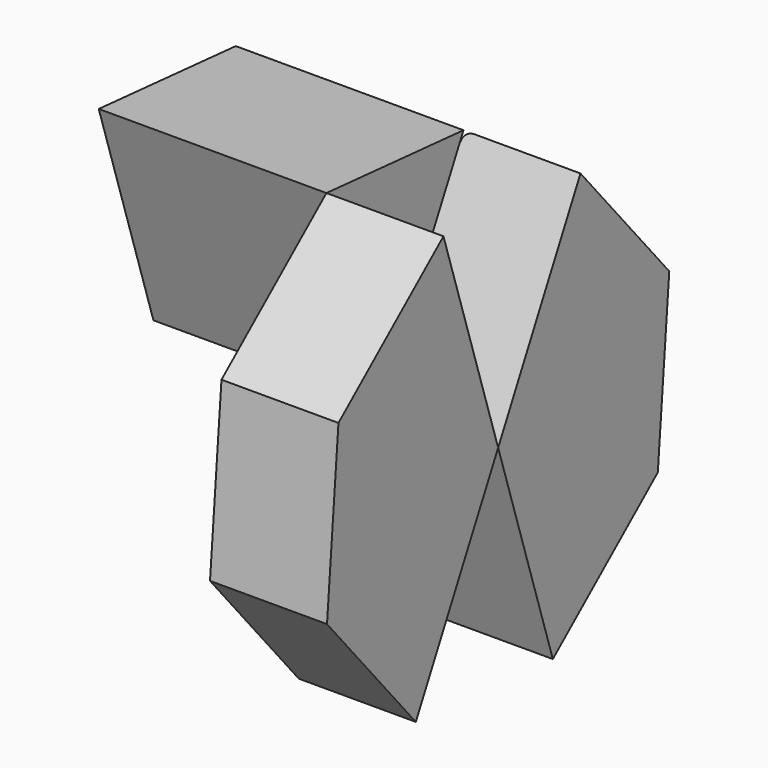
from build123d import *

# Parameters (mm, degrees)
F1_DEPTH     = 12.7
F2_DEPTH     = 25.4
F3_T1_DEPTH  = 25.0079243049
F3_T3_DEPTH  = 25.0079243049
F3_T5_DEPTH  = 25.0079243049
F4_T         = -2.54
F5_T4_DEPTH  = 36.4551670306
F5_T10_DEPTH = 39.8442718127
F5_T16_DEPTH = 39.8442718127
F5_T23_DEPTH = 36.4551670306
F5_T29_DEPTH = 39.8442718127
F5_T38_DEPTH = 36.4551670306
F5_T44_DEPTH = 39.8442718127
F5_T53_DEPTH = 39.8442718127
F5_T59_DEPTH = 39.8442718127


# Not quite as in the source:
# - a fillet or chamfer that OpenCascade refuses, or shapes differently, is made with other operations: its cross-section is extruded or revolved along the edge and cut away or added


with BuildPart() as f1:
    # F0 (on Right) → F1 (new body)
    with BuildSketch(Plane.YZ):
        Polygon((-7.4210610107, 23.220738357), (-21.6670241207, 11.1720589921), (-23.220738357, -7.4210610107), (-11.1720589921, -21.6670241207), (0, 0), align=None)
    extrude(amount=F1_DEPTH)


with BuildPart() as f1b:
    # F0 (on Right) → F1, piece 2 (new body)
    with BuildSketch(Plane.YZ):
        Polygon((23.220738357, 7.4210610107), (11.1720589921, 21.6670241207), (0, 0), (7.4210610107, -23.220738357), (21.6670241207, -11.1720589921), align=None)
    extrude(amount=F1_DEPTH)

    # F3: fillet of radius 1.27 on 3 edges, made by hand

    # F3_s2 → F3_t1 (cut)
    with BuildSketch(Plane(origin=(0, -9.5472026063, -8.074651194), x_dir=(1, 0, 0), z_dir=(0, 0.7635341894, 0.6457674052))):
        with BuildLine():
            add(Edge.make_bspline(
                [(1.27, 22.5221069513), (0, 22.5221069513), (0, 21.2521069513)],
                knots=[0, 0, 0, 1, 1, 1], degree=2, weights=[1, 1, 1]))
            Line((0, 21.2521069513), (0, 22.5221069513))
            Line((0, 22.5221069513), (1.27, 22.5221069513))
        make_face()
    extrude(amount=F3_T1_DEPTH, mode=Mode.SUBTRACT)

    # F3_s4 → F3_t3 (cut)
    with BuildSketch(Plane(origin=(0, -1.0412510893, -12.4605323193), x_dir=(1, 0, 0), z_dir=(0, 0.0832736917, 0.9965267143))):
        with BuildLine():
            add(Edge.make_bspline(
                [(1.27, 22.5221069513), (0, 22.5221069513), (0, 21.2521069513)],
                knots=[0, 0, 0, 1, 1, 1], degree=2, weights=[1, 1, 1]))
            Line((0, 21.2521069513), (0, 22.5221069513))
            Line((0, 22.5221069513), (1.27, 22.5221069513))
        make_face()
    extrude(amount=F3_T3_DEPTH, mode=Mode.SUBTRACT)

    # F3_s6 → F3_t5 (cut)
    with BuildSketch(Plane(origin=(0, 8.074651194, -9.5472026063), x_dir=(1, 0, 0), z_dir=(0, -0.6457674052, 0.7635341894))):
        with BuildLine():
            add(Edge.make_bspline(
                [(1.27, 22.5221069513), (0, 22.5221069513), (0, 21.2521069513)],
                knots=[0, 0, 0, 1, 1, 1], degree=2, weights=[1, 1, 1]))
            Line((0, 21.2521069513), (0, 22.5221069513))
            Line((0, 22.5221069513), (1.27, 22.5221069513))
        make_face()
    extrude(amount=F3_T5_DEPTH, mode=Mode.SUBTRACT)


with BuildPart() as f2:
    # F0 (on Right) → F2 (new body)
    with BuildSketch(Plane.YZ):
        Polygon((11.1720589921, 21.6670241207), (-7.4210610107, 23.220738357), (0, 0), align=None)
    extrude(amount=-F2_DEPTH)

    # F4
    f4_openings = [f2.faces().sort_by_distance(p)[0] for p in [
        (-25.4, 1.250333, 14.962587),
    ]]
    offset(amount=F4_T, openings=f4_openings)

    # F5: fillet of radius 5.08 on 3 edges, made by hand


with BuildPart() as f5_tool2:
    # F5_s3 → F5_t4 (new body)
    with BuildSketch(Plane(origin=(0, 18.1642739097, -1.5178781701), x_dir=(1, 0, 0), z_dir=(0, -0.9965267143, 0.0832736917))):
        with BuildLine():
            ThreePointArc((-25.4, 25.0621069513), (-23.9121024484, 21.4700045029), (-20.32, 19.9821069513))
            Line((-20.32, 19.9821069513), (-25.4, 19.9821069513))
            Line((-25.4, 19.9821069513), (-25.4, 25.0621069513))
        make_face()
    extrude(amount=F5_T4_DEPTH)

    split(bisect_by=Plane(origin=(0, 2.4194467666, 0.7732252864), x_dir=(1, 0, 0), z_dir=(0, 0.9525380971, 0.3044194041)), keep=Keep.TOP)

    split(bisect_by=Plane(origin=(0, -2.2575600588, 1.164054372), x_dir=(1, 0, 0), z_dir=(0, -0.8888031728, 0.4582891228)), keep=Keep.TOP)


with BuildPart() as f2_1:
    add(f2.part)

    # F5_t1: cut F5_tool2
    add(f5_tool2.part, mode=Mode.SUBTRACT)


with BuildPart() as f5_tool8:
    # F5_s9 → F5_t10 (new body)
    with BuildSketch(Plane(origin=(0, -3.0099960077, -5.8375681822), x_dir=(1, 0, 0), z_dir=(0, 0.4582891228, 0.8888031728))):
        with BuildLine():
            ThreePointArc((-25.4, 2.54), (-23.9121024484, -1.0521024484), (-20.32, -2.54))
            Line((-20.32, -2.54), (-25.4, -2.54))
            Line((-25.4, -2.54), (-25.4, 2.54))
        make_face()
    extrude(amount=F5_T10_DEPTH)

    split(bisect_by=Plane(origin=(0, 1.6639838138, 19.9127033846), x_dir=(1, 0, 0), z_dir=(0, -0.0832736917, -0.9965267143)), keep=Keep.TOP)

    split(bisect_by=Plane(origin=(0, 2.4194467666, 0.7732252864), x_dir=(1, 0, 0), z_dir=(0, 0.9525380971, 0.3044194041)), keep=Keep.TOP)


with BuildPart() as f2_2:
    add(f2_1.part)

    # F5_t7: cut F5_tool8
    add(f5_tool8.part, mode=Mode.SUBTRACT)


with BuildPart() as f5_tool14:
    # F5_s15 → F5_t16 (new body)
    with BuildSketch(Plane(origin=(0, -10.1299740234, 31.6970142166), x_dir=(1, 0, 0), z_dir=(0, 0.3044194041, -0.9525380971))):
        with BuildLine():
            ThreePointArc((-25.4, 2.54), (-23.9121024484, -1.0521024484), (-20.32, -2.54))
            Line((-20.32, -2.54), (-25.4, -2.54))
            Line((-25.4, -2.54), (-25.4, 2.54))
        make_face()
    extrude(amount=F5_T16_DEPTH)

    split(bisect_by=Plane(origin=(0, 1.6639838138, 19.9127033846), x_dir=(1, 0, 0), z_dir=(0, -0.0832736917, -0.9965267143)), keep=Keep.TOP)

    split(bisect_by=Plane(origin=(0, -2.2575600588, 1.164054372), x_dir=(1, 0, 0), z_dir=(0, -0.8888031728, 0.4582891228)), keep=Keep.TOP)


with BuildPart() as f2_3:
    add(f2_2.part)

    # F5_t13: cut F5_tool14
    add(f5_tool14.part, mode=Mode.SUBTRACT)


with BuildPart() as f5_tool21:
    # F5_s22 → F5_t23 (new body)
    with BuildSketch(Plane(origin=(0, 18.1642739097, -1.5178781701), x_dir=(1, 0, 0), z_dir=(0, -0.9965267143, 0.0832736917))):
        with BuildLine():
            ThreePointArc((-25.4, 25.0621069513), (-23.9121024484, 21.4700045029), (-20.32, 19.9821069513))
            Line((-20.32, 19.9821069513), (-25.4, 19.9821069513))
            Line((-25.4, 19.9821069513), (-25.4, 25.0621069513))
        make_face()
    extrude(amount=F5_T23_DEPTH)

    split(bisect_by=Plane(origin=(0, 1.8754989907, 22.4438812388), x_dir=(1, 0, 0), z_dir=(0, -0.0832736917, -0.9965267143)), keep=Keep.TOP)

    split(bisect_by=Plane(origin=(0, 0, 0), x_dir=(1, 0, 0), z_dir=(0, -0.8888031728, 0.4582891228)), keep=Keep.TOP)

    split(bisect_by=Plane(origin=(0, -2.2575600588, 1.164054372), x_dir=(1, 0, 0), z_dir=(0, 0.8888031728, -0.4582891228)), keep=Keep.TOP)


with BuildPart() as f5_tool27:
    # F5_s28 → F5_t29 (new body)
    with BuildSketch(Plane(origin=(0, -3.0099960077, -5.8375681822), x_dir=(1, 0, 0), z_dir=(0, 0.4582891228, 0.8888031728))):
        with BuildLine():
            ThreePointArc((-25.4, 2.54), (-23.9121024484, -1.0521024484), (-20.32, -2.54))
            Line((-20.32, -2.54), (-25.4, -2.54))
            Line((-25.4, -2.54), (-25.4, 2.54))
        make_face()
    extrude(amount=F5_T29_DEPTH)

    split(bisect_by=Plane(origin=(0, 1.8754989907, 22.4438812388), x_dir=(1, 0, 0), z_dir=(0, -0.0832736917, -0.9965267143)), keep=Keep.TOP)

    split(bisect_by=Plane(origin=(0, 0, 0), x_dir=(1, 0, 0), z_dir=(0, -0.8888031728, 0.4582891228)), keep=Keep.TOP)

    split(bisect_by=Plane(origin=(0, 1.6639838138, 19.9127033846), x_dir=(1, 0, 0), z_dir=(0, 0.0832736917, 0.9965267143)), keep=Keep.TOP)


with BuildPart() as f5_tool21_1:
    add(f5_tool21.part)

    # F5_t33: intersect F5_tool27
    add(f5_tool27.part, mode=Mode.INTERSECT)


with BuildPart() as f2_4:
    add(f2_3.part)

    # F5_t19: cut F5_tool21
    add(f5_tool21_1.part, mode=Mode.SUBTRACT)


with BuildPart() as f5_tool36:
    # F5_s37 → F5_t38 (new body)
    with BuildSketch(Plane(origin=(0, 18.1642739097, -1.5178781701), x_dir=(1, 0, 0), z_dir=(0, -0.9965267143, 0.0832736917))):
        with BuildLine():
            ThreePointArc((-25.4, 25.0621069513), (-23.9121024484, 21.4700045029), (-20.32, 19.9821069513))
            Line((-20.32, 19.9821069513), (-25.4, 19.9821069513))
            Line((-25.4, 19.9821069513), (-25.4, 25.0621069513))
        make_face()
    extrude(amount=F5_T38_DEPTH)

    split(bisect_by=Plane(origin=(0, 1.8754989907, 22.4438812388), x_dir=(1, 0, 0), z_dir=(0, -0.0832736917, -0.9965267143)), keep=Keep.TOP)

    split(bisect_by=Plane(origin=(0, 0, 0), x_dir=(1, 0, 0), z_dir=(0, 0.9525380971, 0.3044194041)), keep=Keep.TOP)

    split(bisect_by=Plane(origin=(0, 2.4194467666, 0.7732252864), x_dir=(1, 0, 0), z_dir=(0, -0.9525380971, -0.3044194041)), keep=Keep.TOP)


with BuildPart() as f5_tool42:
    # F5_s43 → F5_t44 (new body)
    with BuildSketch(Plane(origin=(0, -10.1299740234, 31.6970142166), x_dir=(1, 0, 0), z_dir=(0, 0.3044194041, -0.9525380971))):
        with BuildLine():
            ThreePointArc((-25.4, 2.54), (-23.9121024484, -1.0521024484), (-20.32, -2.54))
            Line((-20.32, -2.54), (-25.4, -2.54))
            Line((-25.4, -2.54), (-25.4, 2.54))
        make_face()
    extrude(amount=F5_T44_DEPTH)

    split(bisect_by=Plane(origin=(0, 1.8754989907, 22.4438812388), x_dir=(1, 0, 0), z_dir=(0, -0.0832736917, -0.9965267143)), keep=Keep.TOP)

    split(bisect_by=Plane(origin=(0, 0, 0), x_dir=(1, 0, 0), z_dir=(0, 0.9525380971, 0.3044194041)), keep=Keep.TOP)

    split(bisect_by=Plane(origin=(0, 1.6639838138, 19.9127033846), x_dir=(1, 0, 0), z_dir=(0, 0.0832736917, 0.9965267143)), keep=Keep.TOP)


with BuildPart() as f5_tool36_1:
    add(f5_tool36.part)

    # F5_t48: intersect F5_tool42
    add(f5_tool42.part, mode=Mode.INTERSECT)


with BuildPart() as f2_5:
    add(f2_4.part)

    # F5_t34: cut F5_tool36
    add(f5_tool36_1.part, mode=Mode.SUBTRACT)


with BuildPart() as f5_tool51:
    # F5_s52 → F5_t53 (new body)
    with BuildSketch(Plane(origin=(0, -3.0099960077, -5.8375681822), x_dir=(1, 0, 0), z_dir=(0, 0.4582891228, 0.8888031728))):
        with BuildLine():
            ThreePointArc((-25.4, 2.54), (-23.9121024484, -1.0521024484), (-20.32, -2.54))
            Line((-20.32, -2.54), (-25.4, -2.54))
            Line((-25.4, -2.54), (-25.4, 2.54))
        make_face()
    extrude(amount=F5_T53_DEPTH)

    split(bisect_by=Plane(origin=(0, 0, 0), x_dir=(1, 0, 0), z_dir=(0, 0.9525380971, 0.3044194041)), keep=Keep.TOP)

    split(bisect_by=Plane(origin=(0, 0, 0), x_dir=(1, 0, 0), z_dir=(0, -0.8888031728, 0.4582891228)), keep=Keep.TOP)

    split(bisect_by=Plane(origin=(0, 2.4194467666, 0.7732252864), x_dir=(1, 0, 0), z_dir=(0, -0.9525380971, -0.3044194041)), keep=Keep.TOP)


with BuildPart() as f5_tool57:
    # F5_s58 → F5_t59 (new body)
    with BuildSketch(Plane(origin=(0, -10.1299740234, 31.6970142166), x_dir=(1, 0, 0), z_dir=(0, 0.3044194041, -0.9525380971))):
        with BuildLine():
            ThreePointArc((-25.4, 2.54), (-23.9121024484, -1.0521024484), (-20.32, -2.54))
            Line((-20.32, -2.54), (-25.4, -2.54))
            Line((-25.4, -2.54), (-25.4, 2.54))
        make_face()
    extrude(amount=F5_T59_DEPTH)

    split(bisect_by=Plane(origin=(0, 0, 0), x_dir=(1, 0, 0), z_dir=(0, 0.9525380971, 0.3044194041)), keep=Keep.TOP)

    split(bisect_by=Plane(origin=(0, 0, 0), x_dir=(1, 0, 0), z_dir=(0, -0.8888031728, 0.4582891228)), keep=Keep.TOP)

    split(bisect_by=Plane(origin=(0, -2.2575600588, 1.164054372), x_dir=(1, 0, 0), z_dir=(0, 0.8888031728, -0.4582891228)), keep=Keep.TOP)


with BuildPart() as f5_tool51_1:
    add(f5_tool51.part)

    # F5_t63: intersect F5_tool57
    add(f5_tool57.part, mode=Mode.INTERSECT)


with BuildPart() as f2_6:
    add(f2_5.part)

    # F5_t49: cut F5_tool51
    add(f5_tool51_1.part, mode=Mode.SUBTRACT)


solid = Compound([f1.part, f1b.part, f2_6.part])
